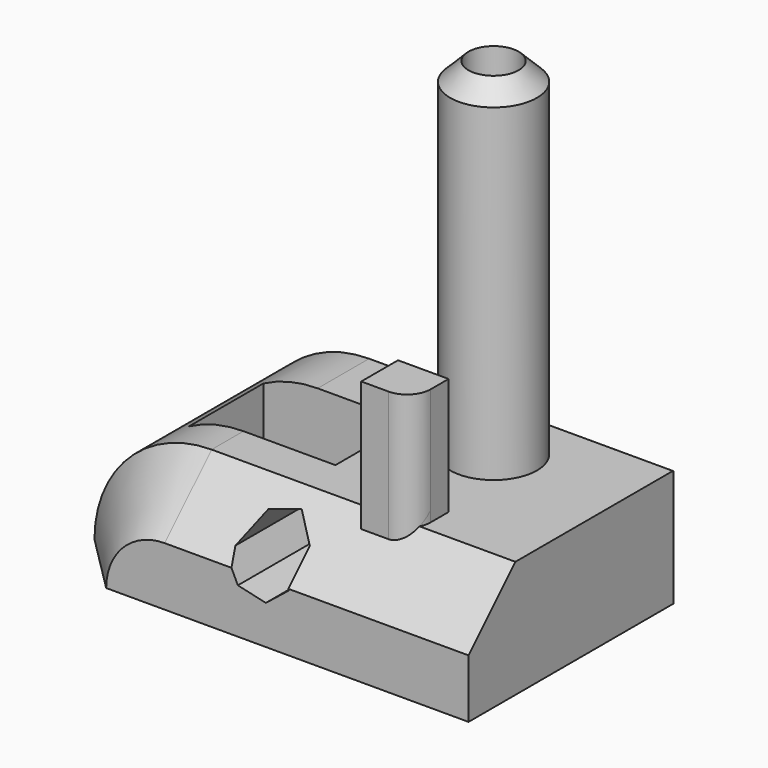
from build123d import *

# Parameters (mm, degrees)
F0_W          = 91.2663862109
F0_H          = 55.5524304509
F1_DEPTH      = 25.4
F2_W          = 31.717389822
F2_H          = 20.1121037826
F3_DEPTH      = 25.401
F4_R          = 9.4254777906
F5_DEPTH      = 76.2
F7_DEPTH      = 55.5534304509
F8_R          = 5.4499976888
F9_DEPTH      = 101.601
F10_W         = 10.9715163708
F10_H         = 9.965904057
F11_DEPTH     = 25.4
F12_T1_DEPTH  = 182.5524304509
F13_T4_DEPTH  = 98.5267601581
F13_T10_DEPTH = 98.5267601581
F13_T16_DEPTH = 98.5267601581
F13_T23_DEPTH = 98.5267601581
F13_T29_DEPTH = 98.5267601581
F13_T33_ANGLE = 163.70288589
F15_T4_DEPTH  = 53.5800548494
F15_T10_DEPTH = 53.5800548494
F15_T16_DEPTH = 53.5800548494
F17_D         = 4.2
F18_R         = 0.254


# Not quite as in the source:
# - a fillet or chamfer that OpenCascade refuses, or shapes differently, is made with other operations: its cross-section is extruded or revolved along the edge and cut away or added


with BuildPart() as f1:
    # F0 (on Top) → F1 (new body)
    with BuildSketch(Plane.XY):
        with Locations((-45.6331931055, -27.7762152255)):
            Rectangle(F0_W, F0_H)
    extrude(amount=F1_DEPTH)

    # F2 (on face) → F3 (cut, through all)
    with BuildSketch(Plane.XY.offset(25.4)):
        with Locations((-61.7938265204, -24.1600726731)):
            Rectangle(F2_W, F2_H)
    extrude(amount=-F3_DEPTH, mode=Mode.SUBTRACT)

    # F4 (on face) → F5 (join)
    with BuildSketch(Plane.XY.offset(25.4)):
        with Locations((-27.4883341044, -14.4118471071)):
            Circle(F4_R)
    extrude(amount=F5_DEPTH)

    # F6 (on face) → F7 (cut, through all)
    with BuildSketch(Plane.XZ.offset(55.5524304509)):
        Polygon((-39.0824638307, 12.301723844), (-39.0824638307, 18.5248410342), (-43.9478927691, 22.4048911381), (-50.0149834187, 21.0201172888), (-52.7150927741, 15.4132824391), (-50.0149834187, 9.8064475894), (-43.9478927691, 8.4216737401), align=None)
    extrude(amount=-F7_DEPTH, mode=Mode.SUBTRACT)

    # F8 (on face) → F9 (cut, through all)
    with BuildSketch(Plane.XY.offset(101.6)):
        with Locations((-27.4883341044, -14.4118471071)):
            Circle(F8_R)
    extrude(amount=-F9_DEPTH, mode=Mode.SUBTRACT)

    # F10 (on face) → F11 (join)
    with BuildSketch(Plane.XY.offset(25.4)):
        with Locations((-25.7194377482, -40.6495332718)):
            Rectangle(F10_W, F10_H)
    extrude(amount=F11_DEPTH)

    # F12: fillet of radius 25.4 on 1 edges, made by hand

    # F12_s2 → F12_t1 (cut)
    with BuildSketch(Plane.XZ.offset(-63.5)):
        with BuildLine():
            ThreePointArc((-91.2663862109, 0), (-83.8268984531, 17.9605122421), (-65.8663862109, 25.4))
            Line((-65.8663862109, 25.4), (-91.2663862109, 25.4))
            Line((-91.2663862109, 25.4), (-91.2663862109, 0))
        make_face()
    extrude(amount=F12_T1_DEPTH, mode=Mode.SUBTRACT)

    # F13: chamfer of 12.7 on 1 edges, made by hand


with BuildPart() as f13_tool2:
    # F13_s3 → F13_t4 (new body)
    with BuildSketch(Plane.YZ.offset(-65.8663862109)):
        Polygon((-55.5524304509, 12.7), (-42.8524304509, 25.4), (-55.5524304509, 25.4), align=None)
    extrude(amount=F13_T4_DEPTH)

    split(bisect_by=Plane.YZ.offset(-31.2051959336), keep=Keep.BOTTOM)

    split(bisect_by=Plane.XZ.offset(45.6324853003), keep=Keep.TOP)


with BuildPart() as f1_1:
    add(f1.part)

    # F13_t1: cut F13_tool2
    add(f13_tool2.part, mode=Mode.SUBTRACT)


with BuildPart() as f13_tool8:
    # F13_s9 → F13_t10 (new body)
    with BuildSketch(Plane.YZ.offset(-65.8663862109)):
        Polygon((-55.5524304509, 12.7), (-42.8524304509, 25.4), (-55.5524304509, 25.4), align=None)
    extrude(amount=F13_T10_DEPTH)

    split(bisect_by=Plane.YZ.offset(-31.2051959336), keep=Keep.BOTTOM)

    split(bisect_by=Plane.XZ.offset(45.6324853003), keep=Keep.BOTTOM)


with BuildPart() as f1_2:
    add(f1_1.part)

    # F13_t7: cut F13_tool8
    add(f13_tool8.part, mode=Mode.SUBTRACT)


with BuildPart() as f13_tool14:
    # F13_s15 → F13_t16 (new body)
    with BuildSketch(Plane.YZ.offset(-65.8663862109)):
        Polygon((-55.5524304509, 12.7), (-42.8524304509, 25.4), (-55.5524304509, 25.4), align=None)
    extrude(amount=F13_T16_DEPTH)

    split(bisect_by=Plane.YZ.offset(-20.2336795628), keep=Keep.BOTTOM)

    split(bisect_by=Plane.YZ.offset(-31.2051959336), keep=Keep.TOP)

    split(bisect_by=Plane.XZ.offset(45.6324853003), keep=Keep.TOP)


with BuildPart() as f1_3:
    add(f1_2.part)

    # F13_t13: cut F13_tool14
    add(f13_tool14.part, mode=Mode.SUBTRACT)


with BuildPart() as f13_tool21:
    # F13_s22 → F13_t23 (new body)
    with BuildSketch(Plane.YZ.offset(-65.8663862109)):
        Polygon((-55.5524304509, 12.7), (-42.8524304509, 25.4), (-55.5524304509, 25.4), align=None)
    extrude(amount=F13_T23_DEPTH)

    split(bisect_by=Plane.YZ.offset(-20.2336795628), keep=Keep.TOP)

    split(bisect_by=Plane.XZ.offset(45.6324853003), keep=Keep.TOP)


with BuildPart() as f1_4:
    add(f1_3.part)

    # F13_t20: cut F13_tool21
    add(f13_tool21.part, mode=Mode.SUBTRACT)


with BuildPart() as f13_tool27:
    # F13_s28 → F13_t29 (new body)
    with BuildSketch(Plane.YZ.offset(-65.8663862109)):
        Polygon((-55.5524304509, 12.7), (-42.8524304509, 25.4), (-55.5524304509, 25.4), align=None)
    extrude(amount=F13_T29_DEPTH)

    split(bisect_by=Plane.YZ.offset(-20.2336795628), keep=Keep.TOP)

    split(bisect_by=Plane.XZ.offset(45.6324853003), keep=Keep.BOTTOM)


with BuildPart() as f1_5:
    add(f1_4.part)

    # F13_t26: cut F13_tool27
    add(f13_tool27.part, mode=Mode.SUBTRACT)

    # F13_s32 → F13_t33 (revolve, cut)
    with BuildSketch(Plane(origin=(-60.6796278509, 0, 17.7406473118), x_dir=(0, 1, 0), z_dir=(0.9598194275, 0, -0.2806183648))):
        Polygon((-42.8524304509, -43.8833175952), (-55.5524304509, -31.1833175952), (-55.5524304509, -43.8833175952), align=None)
    revolve(axis=Axis((-65.8663862109, -55.5524304509, 0), (0, 1, 0)), revolution_arc=F13_T33_ANGLE, mode=Mode.SUBTRACT)

    # F14: chamfer of 5.08 on 1 edges, made by hand

    # F14_s1 → F14_t2 (revolve, cut)
    with BuildSketch(Plane.XZ.offset(14.4118471071)):
        Polygon((-23.1428563138, 101.6), (-18.0628563138, 96.52), (-18.0628563138, 101.6), align=None)
    revolve(axis=Axis((-27.4883341044, -14.4118471071, 101.6), (0, 0, 1)), mode=Mode.SUBTRACT)

    # F15: fillet of radius 5.08 on 1 edges, made by hand


with BuildPart() as f15_tool2:
    # F15_s3 → F15_t4 (new body)
    with BuildSketch(Plane.XY.offset(63.5)):
        with BuildLine():
            ThreePointArc((-20.2336795628, -40.5524853003), (-21.7215771144, -44.1445877487), (-25.3136795628, -45.6324853003))
            Line((-25.3136795628, -45.6324853003), (-20.2336795628, -45.6324853003))
            Line((-20.2336795628, -45.6324853003), (-20.2336795628, -40.5524853003))
        make_face()
    extrude(amount=-F15_T4_DEPTH)

    split(bisect_by=Plane.XY.offset(25.4), keep=Keep.TOP)

    split(bisect_by=Plane(origin=(0, -34.1262152254, 34.1262152254), x_dir=(1, 0, 0), z_dir=(0, -0.7071067812, 0.7071067812)), keep=Keep.TOP)


with BuildPart() as f1_6:
    add(f1_5.part)

    # F15_t1: cut F15_tool2
    add(f15_tool2.part, mode=Mode.SUBTRACT)


with BuildPart() as f15_tool8:
    # F15_s9 → F15_t10 (new body)
    with BuildSketch(Plane.XY.offset(63.5)):
        with BuildLine():
            ThreePointArc((-20.2336795628, -40.5524853003), (-21.7215771144, -44.1445877487), (-25.3136795628, -45.6324853003))
            Line((-25.3136795628, -45.6324853003), (-20.2336795628, -45.6324853003))
            Line((-20.2336795628, -45.6324853003), (-20.2336795628, -40.5524853003))
        make_face()
    extrude(amount=-F15_T10_DEPTH)

    split(bisect_by=Plane.XY.offset(25.4), keep=Keep.BOTTOM)

    split(bisect_by=Plane(origin=(0, -34.1262152255, 34.1262152254), x_dir=(1, 0, 0), z_dir=(0, -0.7071067812, 0.7071067812)), keep=Keep.TOP)


with BuildPart() as f1_7:
    add(f1_6.part)

    # F15_t7: cut F15_tool8
    add(f15_tool8.part, mode=Mode.SUBTRACT)


with BuildPart() as f15_tool14:
    # F15_s15 → F15_t16 (new body)
    with BuildSketch(Plane.XY.offset(63.5)):
        with BuildLine():
            ThreePointArc((-20.2336795628, -40.5524853003), (-21.7215771144, -44.1445877487), (-25.3136795628, -45.6324853003))
            Line((-25.3136795628, -45.6324853003), (-20.2336795628, -45.6324853003))
            Line((-20.2336795628, -45.6324853003), (-20.2336795628, -40.5524853003))
        make_face()
    extrude(amount=-F15_T16_DEPTH)

    split(bisect_by=Plane.XY.offset(25.4), keep=Keep.TOP)

    split(bisect_by=Plane(origin=(0, -34.1262152255, 34.1262152254), x_dir=(1, 0, 0), z_dir=(0, 0.7071067812, -0.7071067812)), keep=Keep.TOP)


with BuildPart() as f1_8:
    add(f1_7.part)

    # F15_t13: cut F15_tool14
    add(f15_tool14.part, mode=Mode.SUBTRACT)

    # F17 (through all)
    with Locations(Plane.XY.offset(25.4)):
        with Locations((-37.6806370914, -34.2161245644), (-43.5164868832, -5.5432366207)):
            Hole(F17_D / 2)

    # F18
    f18_edges = [f1_8.edges().sort_by_distance(p)[0] for p in [
        (-83.826898, 0, 17.960512),
    ]]
    fillet(f18_edges, radius=F18_R)


solid = f1_8.part
